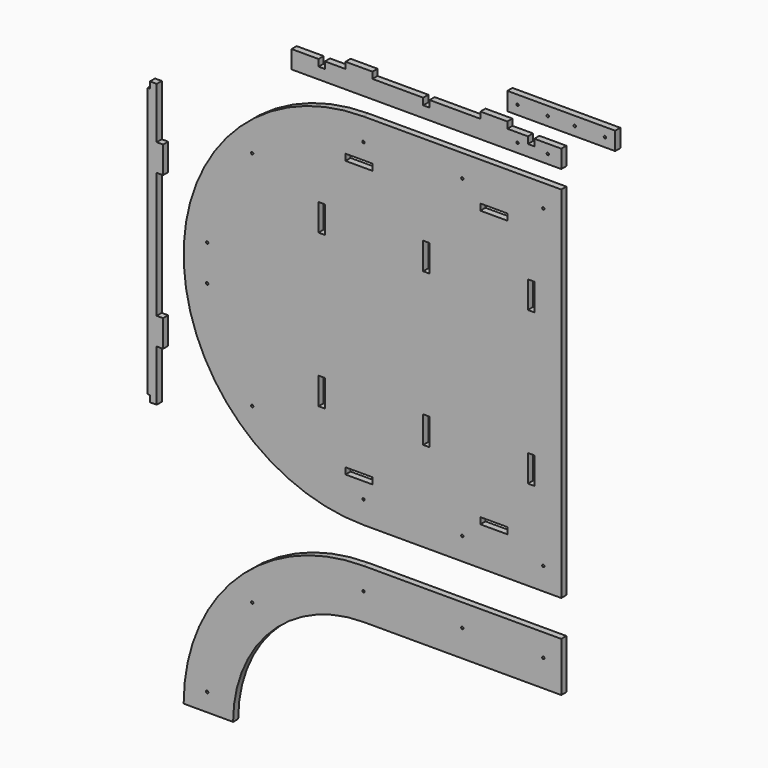
from build123d import *

# Parameters (mm, degrees)
F1_W     = 19.05
F1_H     = 18.034
F1_W_2   = 18.034
F1_H_2   = 76.2
F2_DEPTH = 18.034
F1_R     = 3.302
F1_W_3   = 76.2
F1_W_4   = 304.8
F1_H_3   = 50.8


# Not quite as in the source:
# - a variable given as a bare number and used for a length is read in inches; the dataset says mm whatever the document's units were


with BuildPart() as f2:
    # F1 (on Front) → F2 (new body)
    with BuildSketch(Plane.XZ):
        with Locations((-1152.525, 390.017)):
            Rectangle(F1_W, F1_H)
        Polygon((-1162.05, -381), (-1143, -381), (-1143, -254), (-1143, -177.8), (-1143, 177.8), (-1143, 254), (-1143, 381), (-1162.05, 381), (-1168.4, 381), (-1168.4, -381), align=None)
        with Locations((-1133.983, 215.9)):
            Rectangle(F1_W_2, F1_H_2)
        with Locations((-1152.525, -390.017)):
            Rectangle(F1_W, F1_H)
        with Locations((-1133.983, -215.9)):
            Rectangle(F1_W_2, F1_H_2)
    extrude(amount=F2_DEPTH)


with BuildPart() as f2b:
    # F1 (on Front) → F2, piece 2 (new body)
    with BuildSketch(Plane.XZ):
        with BuildLine():
            Line((0, -508), (0, 508))
            Line((0, 508), (-558.8, 508))
            ThreePointArc((-558.8, 508), (-1066.8, 0), (-558.8, -508))
            Line((-558.8, -508), (0, -508))
        make_face()
        with Locations((-873.1089642374, -314.3089642374)):
            Circle(F1_R, mode=Mode.SUBTRACT)
        with Locations((-558.8, -444.5)):
            Circle(F1_R, mode=Mode.SUBTRACT)
        with Locations((-676.783, -215.9)):
            Rectangle(F1_W_2, F1_H_2, mode=Mode.SUBTRACT)
        with Locations((-571.5, -390.017)):
            Rectangle(F1_W_3, F1_H, mode=Mode.SUBTRACT)
        with Locations((-279.4, -444.5)):
            Circle(F1_R, mode=Mode.SUBTRACT)
        with Locations((-381, -215.9)):
            Rectangle(F1_W_2, F1_H_2, mode=Mode.SUBTRACT)
        with Locations((-190.5, -390.017)):
            Rectangle(F1_W_3, F1_H, mode=Mode.SUBTRACT)
        with Locations((-50.8, -444.5)):
            Circle(F1_R, mode=Mode.SUBTRACT)
        with Locations((-85.217, -215.9)):
            Rectangle(F1_W_2, F1_H_2, mode=Mode.SUBTRACT)
        with Locations((-1000.3876017281, -50.8)):
            Circle(F1_R, mode=Mode.SUBTRACT)
        with Locations((-1000.3876017281, 50.8)):
            Circle(F1_R, mode=Mode.SUBTRACT)
        with Locations((-676.783, 215.9)):
            Rectangle(F1_W_2, F1_H_2, mode=Mode.SUBTRACT)
        with Locations((-873.1089642374, 314.3089642374)):
            Circle(F1_R, mode=Mode.SUBTRACT)
        with Locations((-571.5, 390.017)):
            Rectangle(F1_W_3, F1_H, mode=Mode.SUBTRACT)
        with Locations((-558.8, 444.5)):
            Circle(F1_R, mode=Mode.SUBTRACT)
        with Locations((-381, 215.9)):
            Rectangle(F1_W_2, F1_H_2, mode=Mode.SUBTRACT)
        with Locations((-85.217, 215.9)):
            Rectangle(F1_W_2, F1_H_2, mode=Mode.SUBTRACT)
        with Locations((-279.4, 444.5)):
            Circle(F1_R, mode=Mode.SUBTRACT)
        with Locations((-190.5, 390.017)):
            Rectangle(F1_W_3, F1_H, mode=Mode.SUBTRACT)
        with Locations((-50.8, 444.5)):
            Circle(F1_R, mode=Mode.SUBTRACT)
    extrude(amount=F2_DEPTH)


with BuildPart() as f2c:
    # F1 (on Front) → F2, piece 3 (new body)
    with BuildSketch(Plane.XZ):
        with BuildLine():
            Line((0, -749.3), (0, -609.6))
            Line((0, -609.6), (-558.8, -609.6))
            ThreePointArc((-558.8, -609.6), (-918.0102448428, -758.3897551572), (-1066.8, -1117.6))
            Line((-1066.8, -1117.6), (-927.1, -1117.6))
            ThreePointArc((-927.1, -1117.6), (-819.227427511, -857.172572489), (-558.8, -749.3))
            Line((-558.8, -749.3), (0, -749.3))
        make_face()
        with Locations((-1000.3876017281, -1066.8)):
            Circle(F1_R, mode=Mode.SUBTRACT)
        with Locations((-873.1089642374, -803.2910357626)):
            Circle(F1_R, mode=Mode.SUBTRACT)
        with Locations((-558.8, -673.1)):
            Circle(F1_R, mode=Mode.SUBTRACT)
        with Locations((-279.4, -673.1)):
            Circle(F1_R, mode=Mode.SUBTRACT)
        with Locations((-50.8, -673.1)):
            Circle(F1_R, mode=Mode.SUBTRACT)
    extrude(amount=F2_DEPTH)


with BuildPart() as f2d:
    # F1 (on Front) → F2, piece 4 (new body)
    with BuildSketch(Plane.XZ):
        Polygon((-762, 609.6), (-762, 558.8), (0, 558.8), (0, 609.6), (-76.2, 609.6), (-76.2, 590.55), (-94.234, 590.55), (-94.234, 609.6), (-152.4, 609.6), (-228.6, 609.6), (-371.983, 609.6), (-371.983, 590.55), (-390.017, 590.55), (-390.017, 609.6), (-533.4, 609.6), (-609.6, 609.6), (-667.766, 609.6), (-667.766, 590.55), (-685.8, 590.55), (-685.8, 609.6), align=None)
        with Locations((-123.317, 584.2)):
            Circle(F1_R, mode=Mode.SUBTRACT)
        with Locations((-38.1, 584.2)):
            Circle(F1_R, mode=Mode.SUBTRACT)
        with Locations((-571.5, 618.617)):
            Rectangle(F1_W_3, F1_H)
        with Locations((-190.5, 618.617)):
            Rectangle(F1_W_3, F1_H)
    extrude(amount=F2_DEPTH)


with BuildPart() as f2e:
    # F1 (on Front) → F2, piece 5 (new body)
    with BuildSketch(Plane.XZ):
        with Locations((0, 678.434)):
            Rectangle(F1_W_4, F1_H_3)
        with Locations((-123.317, 678.434)):
            Circle(F1_R, mode=Mode.SUBTRACT)
        with Locations((-38.1, 678.434)):
            Circle(F1_R, mode=Mode.SUBTRACT)
        with Locations((38.1, 678.434)):
            Circle(F1_R, mode=Mode.SUBTRACT)
        with Locations((123.317, 678.434)):
            Circle(F1_R, mode=Mode.SUBTRACT)
    extrude(amount=F2_DEPTH)


solid = Compound([f2.part, f2b.part, f2c.part, f2d.part, f2e.part])
